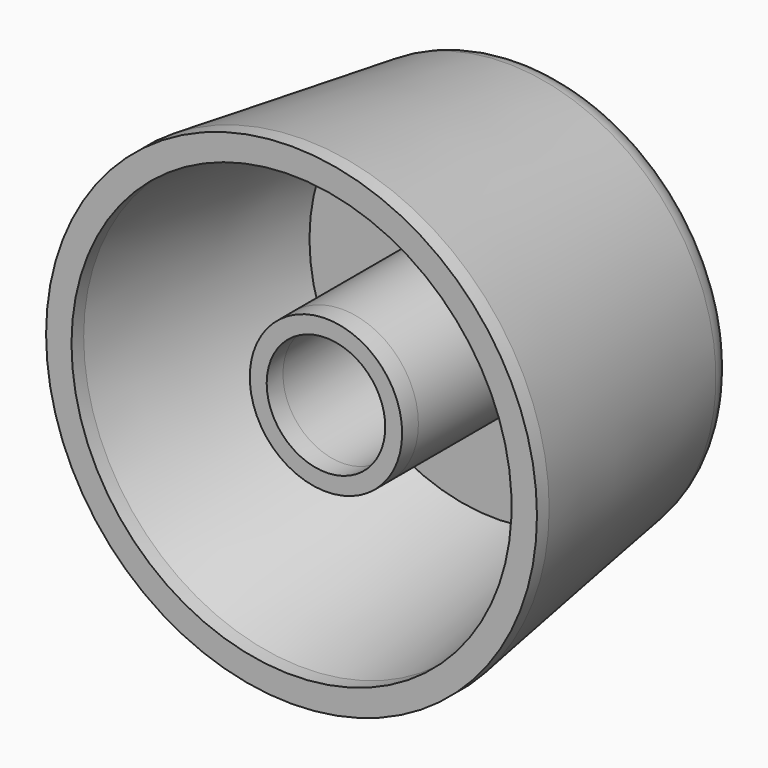
from build123d import *
from build123d import SkipClean  # not in build123d's __all__

# Parameters (mm, degrees)
F2_R     = 2
F4_DEPTH = 6
F5_DEPTH = 10
F6_DEPTH = 0.9
F3_R     = 4.4988269867
F7_DEPTH = 1.2


with BuildPart() as f1:
    # F0 (on Top) → F1 (revolve)
    with BuildSketch(Plane.XY):
        Polygon((0.6408938694, 2.8410089679), (0.6408938694, 16.7043862722), (-11.46528483, 16.7043862722), (-13.8516243371, 0), (-12.3516243371, 0), (-10.3318675491, 14.1383057447), (-3.8579331173, 14.1383057447), (-3.8579331173, 2.8410089679), align=None)
    revolve(axis=Axis((0.6408938694, 3.1900271702, 0), (0, -1, 0)))

    # F2
    f2_edges = [f1.edges().sort_by_distance(p)[0] for p in [
        (12.747073, 16.704386, 0),
    ]]
    fillet(f2_edges, radius=F2_R)

    # F3 (on face) → F4 (cut)
    with BuildSketch(Plane.XZ.offset(-2.8410089679)):
        with BuildLine():
            ThreePointArc((3.3910251828, -2.1648967087), (3.9481177503, -1.1455436271), (4.1408938694, 0))
            ThreePointArc((4.1408938694, 0), (3.9481177503, 1.1455436271), (3.3910251828, 2.1648967087))
            Line((3.3910251828, 2.1648967087), (3.3910251828, -2.1648967087))
        make_face()
        with BuildLine():
            Line((3.3910251828, -2.1648967087), (3.3910251828, 2.1648967087))
            ThreePointArc((3.3910251828, 2.1648967087), (-2.8591061306, 0), (3.3910251828, -2.1648967087))
        make_face()
    extrude(amount=-F4_DEPTH, mode=Mode.SUBTRACT)

    # F3 (on face) → F5 (cut)
    with BuildSketch(Plane.XZ.offset(-2.8410089679)):
        with BuildLine():
            Line((3.3910251828, -2.1648967087), (3.3910251828, 2.1648967087))
            ThreePointArc((3.3910251828, 2.1648967087), (-2.8591061306, 0), (3.3910251828, -2.1648967087))
        make_face()
    extrude(amount=-F5_DEPTH, mode=Mode.SUBTRACT)

    # F6 (add): a face of the model
    f6_faces = [f1.faces().sort_by_distance(p)[0] for p in [
        (14.72350176, 0, 0),
    ]]
    extrude(f6_faces, amount=F6_DEPTH)

    # F3 (on face) → F7 (join)
    with BuildSketch(Plane.XZ.offset(-2.8410089679)):
        with Locations((0.6408938694, 0)):
            Circle(F3_R)
        with BuildLine():
            ThreePointArc((3.3910251828, 2.1648967087), (3.9481177503, 1.1455436271), (4.1408938694, 0))
            ThreePointArc((4.1408938694, 0), (3.9481177503, -1.1455436271), (3.3910251828, -2.1648967087))
            ThreePointArc((3.3910251828, -2.1648967087), (-2.8591061306, 0), (3.3910251828, 2.1648967087))
        make_face(mode=Mode.SUBTRACT)
    with SkipClean():  # cleaning this boolean's faces spoils the solid; the shape is the same uncleaned
        extrude(amount=F7_DEPTH)


solid = f1.part
